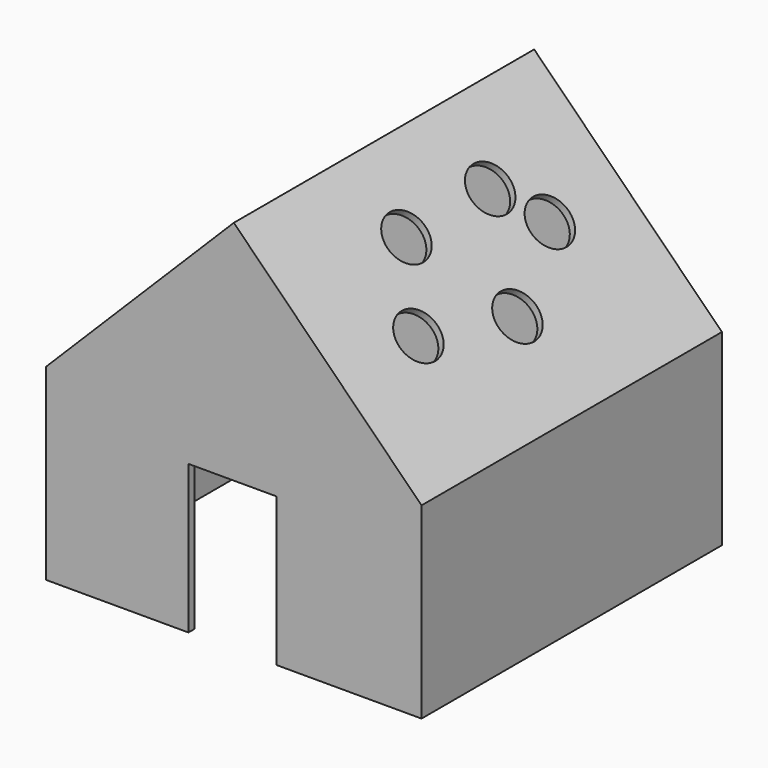
from build123d import *

# Parameters (mm, degrees)
F0_W     = 100
F0_H     = 100
F1_DEPTH = 100
F2_SIZE2 = 49.99999
F2_SIZE  = 49.99999
F3_T     = -2
F4_W     = 23.5146284103
F4_H     = 39.5418182015
F5_DEPTH = 2
F7_D     = 12.6
F7_DEPTH = 17.25
F7_TIP   = 3.7854218999


# Not quite as in the source:
# - a fillet or chamfer is up to 0.001 mm smaller than in the source, because OpenCascade refuses the exact size


with BuildPart() as f1:
    # F0 (on Top) → F1 (new body)
    with BuildSketch(Plane.XY):
        Rectangle(F0_W, F0_H)
    extrude(amount=F1_DEPTH)

    # F2 (size 50 and 50 in the source; OpenCascade refuses exactly that, so slightly less here)
    f2_edges = [f1.edges().sort_by_distance(p)[0] for p in [
        (-50, 0, 100),
        (50, 0, 100),
    ]]
    chamfer(f2_edges, length=F2_SIZE, length2=F2_SIZE2)

    # F3
    f3_openings = [f1.faces().sort_by_distance(p)[0] for p in [
        (0, 0, 0),
    ]]
    offset(amount=F3_T, openings=f3_openings)

    # F4 (on face) → F5 (cut, through all)
    with BuildSketch(Plane.XZ.offset(50)):
        with Locations((-0.3359224647, 19.7709091008)):
            Rectangle(F4_W, F4_H)
    extrude(amount=-F5_DEPTH, mode=Mode.SUBTRACT)

    # F7
    with Locations(Plane(origin=(50, 0, 50), x_dir=(0, 1, 0), z_dir=(0.7071067812, 0, 0.7071067812))):
        with Locations((17.1098317951, 50.0659272075), (-10.7799200341, 50.0659272075), (-23.6778985709, 30.9631545097), (3.2679832075, 24.1581760347), (26.1959340423, 37.8756783903)):
            Hole(F7_D / 2, depth=F7_DEPTH)
            with Locations((0, 0, -(F7_DEPTH + F7_TIP / 2))):  # 118° drill point
                Cone(0, F7_D / 2, F7_TIP, mode=Mode.SUBTRACT)


solid = f1.part
